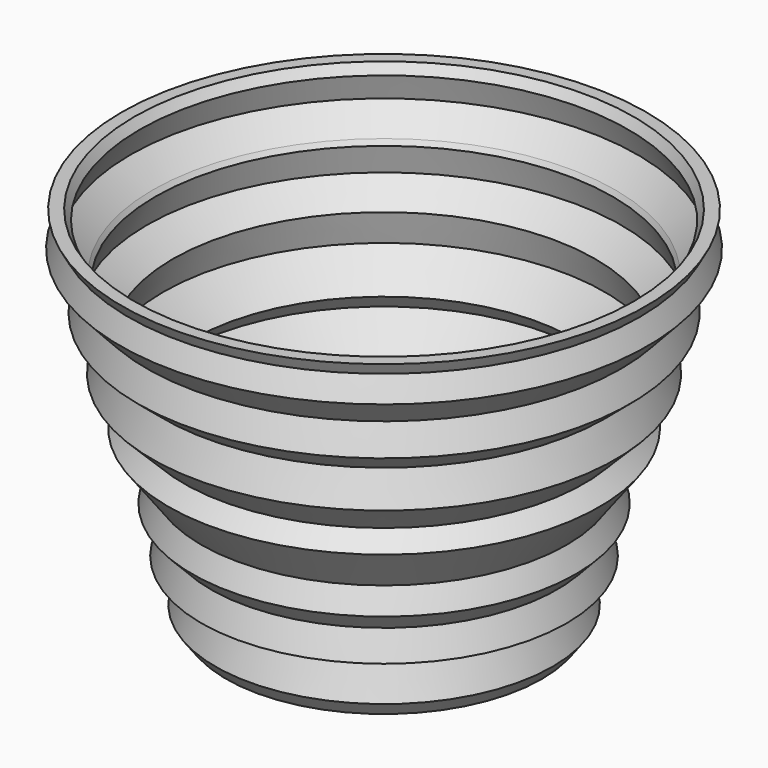
from build123d import *

# Parameters (mm, degrees)
F2_TEXT_SIZE = 9.3290747221
F3_DEPTH     = 1.8611927525


# Not quite as in the source:
# - Text() gives the source's letters only with a copy of the font that has no kerning and outlines rounded to 1/6400 em; it was checked with that copy


with BuildPart() as f1:
    # F0 (on Front) → F1 (revolve)
    with BuildSketch(Plane.XZ):
        Polygon((-32.4877873063, 47.1224561334), (-34.1146923602, 47.1224561334), (-33.2530066371, 45.5683916807), (-34.3235768378, 42.6243208349), (-30.8442227542, 38.8773232698), (-32.048612833, 35.2641455829), (-28.7030804902, 32.4538983405), (-30.1751140505, 28.3054374158), (-26.0266531259, 24.1569746286), (-28.0339740998, 22.1496545559), (-23.7516891211, 16.395336017), (-24.9560810626, 13.4512661025), (-22.5472971797, 10.9086604789), (-23.7516891211, 7.4268425815), (-20.3950445146, 6.2657492005), (-21.9189658798, 1.8601927525), (-20.5346359322, 0), (0, 0), (0, 1.8601927525), (-20.0465840515, 1.8601927525), (-18.5780682637, 6.2657492005), (-19.2218624048, 7.4268425815), (-21.6479099371, 8.2355234247), (-20.7568660898, 10.9086604789), (-23.2994705717, 13.4512661025), (-22.2548012843, 16.395336017), (-26.537086263, 22.1496545559), (-24.8509373573, 24.1569746286), (-28.7030804902, 28.3054374158), (-27.4986904114, 32.4538983405), (-30.8442227542, 35.2641455829), (-29.7385764766, 38.8773232698), (-30.0970124932, 39.5237685538), (-32.9760960936, 42.6243208349), (-31.7948540483, 45.8727395424), align=None)
    revolve(axis=Axis((0, 0, 25.133907795), (0, 0, -1)))

    # F2 (on face) → F3 (cut, through all)
    with BuildSketch(Plane.XY.offset(1.8601927525)):
        with Locations((-14.6525399759, -3.2452782616)):
            Text('Iceman', F2_TEXT_SIZE, font='Open Sans', font_style=FontStyle.ITALIC, text_align=(TextAlign.LEFT, TextAlign.BOTTOM))
    extrude(amount=-F3_DEPTH, mode=Mode.SUBTRACT)


solid = f1.part
